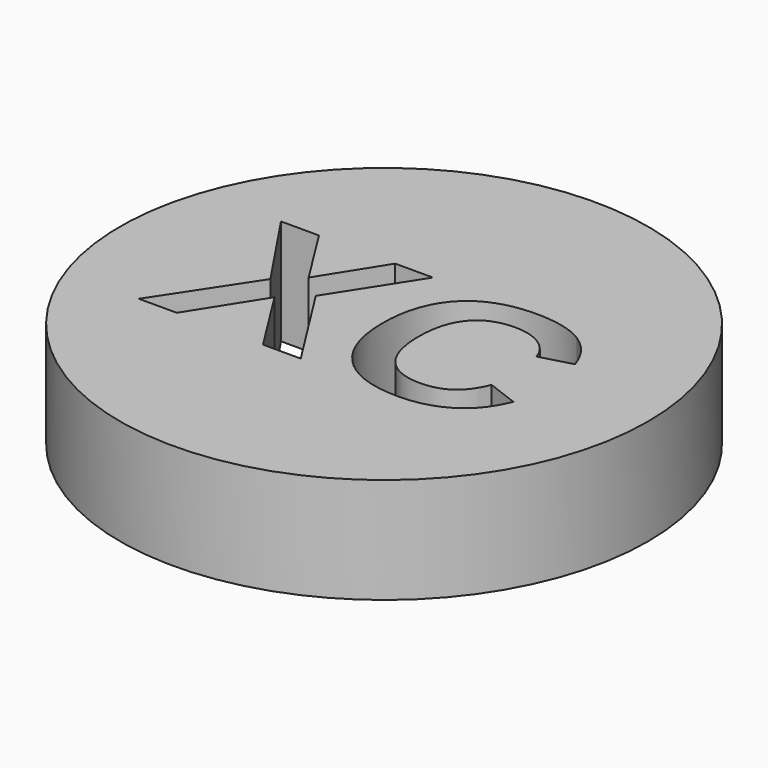
from build123d import *

# Parameters (mm, degrees)
F0_R     = 25
F1_DEPTH = 10


with BuildPart() as f1:
    # F0 (on Top) → F1 (new body)
    with BuildSketch(Plane.XY):
        Circle(F0_R)
        Polygon((-1.3539496528, -8.1774380319), (-4.9288194444, -8.1774380319), (-9.0091145833, -1.7102071291), (-13.0930989583, -8.1774380319), (-16.6901041667, -8.1774380319), (-11.0640190972, 0.3668328015), (-16.2178819444, 8.0662685653), (-12.6208767361, 8.0662685653), (-9.0091145833, 2.3258171765), (-5.4010416667, 8.0662685653), (-1.8298611111, 8.0662685653), (-6.7623697917, 0.3668328015), align=None, mode=Mode.SUBTRACT)
        with BuildLine():
            add(Edge.make_bspline(
                [(4.4731987847, -4.2557800458), (5.6998697917, -5.7314744902), (8.0167100694, -5.7314744902)],
                knots=[0, 0, 0, 1, 1, 1], degree=2))
            add(Edge.make_bspline(
                [(8.0167100694, -5.7314744902), (11.0972222222, -5.7314744902), (12.2962239583, -2.6435838652)],
                knots=[0, 0, 0, 1, 1, 1], degree=2))
            Line((12.2962239583, -2.6435838652), (15.2586805556, -3.7614224069))
            add(Edge.make_bspline(
                [(15.2586805556, -3.7614224069), (14.3031684028, -6.1151550458), (12.451171875, -7.2625074763)],
                knots=[0, 0, 0, 1, 1, 1], degree=2))
            add(Edge.make_bspline(
                [(12.451171875, -7.2625074763), (10.5991753472, -8.4098599069), (8.0167100694, -8.4098599069)],
                knots=[0, 0, 0, 1, 1, 1], degree=2))
            add(Edge.make_bspline(
                [(8.0167100694, -8.4098599069), (4.0987413194, -8.4098599069), (1.9608289931, -6.188939768)],
                knots=[0, 0, 0, 1, 1, 1], degree=2))
            add(Edge.make_bspline(
                [(1.9608289931, -6.188939768), (-0.1770833333, -3.9680196291), (-0.1770833333, 0.020044607)],
                knots=[0, 0, 0, 1, 1, 1], degree=2))
            add(Edge.make_bspline(
                [(-0.1770833333, 0.020044607), (-0.1770833333, 4.0191765515), (1.8851996528, 6.1644673501)],
                knots=[0, 0, 0, 1, 1, 1], degree=2))
            add(Edge.make_bspline(
                [(1.8851996528, 6.1644673501), (3.9474826389, 8.3097581487), (7.869140625, 8.3097581487)],
                knots=[0, 0, 0, 1, 1, 1], degree=2))
            add(Edge.make_bspline(
                [(7.869140625, 8.3097581487), (10.7282986111, 8.3097581487), (12.5268012153, 7.1624057181)],
                knots=[0, 0, 0, 1, 1, 1], degree=2))
            add(Edge.make_bspline(
                [(12.5268012153, 7.1624057181), (14.3253038194, 6.0150532876), (15.0520833333, 3.7904439126)],
                knots=[0, 0, 0, 1, 1, 1], degree=2))
            Line((15.0520833333, 3.7904439126), (12.052734375, 2.9714334959))
            add(Edge.make_bspline(
                [(12.052734375, 2.9714334959), (11.6727430556, 4.1925706487), (10.5604383681, 4.9138163084)],
                knots=[0, 0, 0, 1, 1, 1], degree=2))
            add(Edge.make_bspline(
                [(10.5604383681, 4.9138163084), (9.4481336806, 5.6350619681), (7.9392361111, 5.6350619681)],
                knots=[0, 0, 0, 1, 1, 1], degree=2))
            add(Edge.make_bspline(
                [(7.9392361111, 5.6350619681), (5.6334635417, 5.6350619681), (4.4399956597, 4.2054829751)],
                knots=[0, 0, 0, 1, 1, 1], degree=2))
            add(Edge.make_bspline(
                [(4.4399956597, 4.2054829751), (3.2465277778, 2.775903982), (3.2465277778, 0.020044607)],
                knots=[0, 0, 0, 1, 1, 1], degree=2))
            add(Edge.make_bspline(
                [(3.2465277778, 0.020044607), (3.2465277778, -2.7800856013), (4.4731987847, -4.2557800458)],
                knots=[0, 0, 0, 1, 1, 1], degree=2))
        make_face(mode=Mode.SUBTRACT)
    extrude(amount=F1_DEPTH)


solid = f1.part
